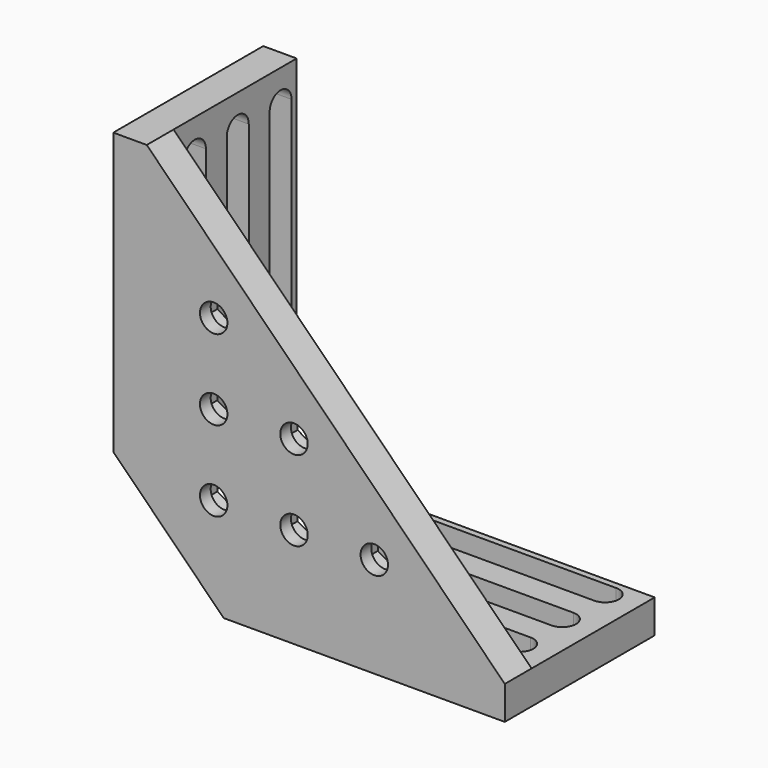
from build123d import *

# Parameters (mm, degrees)
F0_W      = 42
F0_H      = 23
F1_DEPTH  = 5
F3_ANGLE  = 90
F8_R      = 2.05
F9_DEPTH  = 5
F10_DEPTH = 3


# Not quite as in the source:
# - a feature names something its author has since deleted; it is built from what else it names


with BuildPart() as f1:
    # F0 (on Top) → F1 (new body)
    with BuildSketch(Plane.XY):
        Rectangle(F0_W, F0_H)
        with BuildLine():
            ThreePointArc((-16, -9.55), (-18.05, -7.5), (-16, -5.45))
            Line((-16, -5.45), (16, -5.45))
            ThreePointArc((16, -5.45), (18.05, -7.5), (16, -9.55))
            Line((16, -9.55), (-16, -9.55))
        make_face(mode=Mode.SUBTRACT)
        with BuildLine():
            Line((0, -1.55), (-16, -1.55))
            ThreePointArc((-16, -1.55), (-18.05, 0.5), (-16, 2.55))
            Line((-16, 2.55), (0, 2.55))
            Line((0, 2.55), (16, 2.55))
            ThreePointArc((16, 2.55), (18.05, 0.5), (16, -1.55))
            Line((16, -1.55), (0, -1.55))
        make_face(mode=Mode.SUBTRACT)
        with BuildLine():
            Line((16, 6.45), (-16, 6.45))
            ThreePointArc((-16, 6.45), (-18.05, 8.5), (-16, 10.55))
            Line((-16, 10.55), (16, 10.55))
            ThreePointArc((16, 10.55), (18.05, 8.5), (16, 6.45))
        make_face(mode=Mode.SUBTRACT)
    extrude(amount=F1_DEPTH)


with BuildPart() as f3_1:
    # F3: copy of F1
    add(f1.part.rotate(Axis((-21, 0, 2.5), (0, -1, 0)), F3_ANGLE))


with BuildPart() as f3_1_1:
    # F4: moved
    add(f3_1.part.moved(Location((0, 0, 14))))


with BuildPart() as f3_1_2:
    # F5: moved
    add(f3_1_1.part.moved(Location((-14, 0, 0))))


with BuildPart() as f1_1:
    add(f1.part)

    add(f3_1_2.part)  # F9 merges F3_1
    # F8 (on 3pt) → F9 (join)
    with BuildSketch(Plane.XZ.offset(11.5)):
        Polygon((-37.5, 16.5), (-21, 0), (21, 0), (21, 5), (14.4509618943, 11.5490381057), (13.5, 11), (10.0358983849, 13), (10.0358983849, 15.9641016151), (2.4509618943, 23.5490381057), (1.5, 23), (-1.9641016151, 25), (-1.9641016151, 27.9641016151), (-9.5490381057, 35.5490381057), (-10.5, 35), (-13.9641016151, 37), (-13.9641016151, 39.9641016151), (-21.5490381057, 47.5490381057), (-22.5, 47), (-25.9641016151, 49), (-25.9641016151, 51.9641016151), (-32.5, 58.5), (-37.5, 58.5), align=None)
        Polygon((-25.9641016151, 17), (-22.5, 19), (-19.0358983849, 17), (-19.0358983849, 13), (-22.5, 11), (-25.9641016151, 13), align=None, mode=Mode.SUBTRACT)
        Polygon((-13.9641016151, 13), (-13.9641016151, 17), (-10.5, 19), (-7.0358983849, 17), (-7.0358983849, 13), (-10.5, 11), align=None, mode=Mode.SUBTRACT)
        Polygon((-25.9641016151, 25), (-25.9641016151, 29), (-22.5, 31), (-19.0358983849, 29), (-19.0358983849, 25), (-22.5, 23), align=None, mode=Mode.SUBTRACT)
        Polygon((-13.9641016151, 25), (-13.9641016151, 29), (-10.5, 31), (-7.0358983849, 29), (-7.0358983849, 25), (-10.5, 23), align=None, mode=Mode.SUBTRACT)
        Polygon((-1.9641016151, 13), (-1.9641016151, 17), (1.5, 19), (4.9641016151, 17), (4.9641016151, 13), (1.5, 11), align=None, mode=Mode.SUBTRACT)
        Polygon((-25.9641016151, 37), (-25.9641016151, 41), (-22.5, 43), (-19.0358983849, 41), (-19.0358983849, 37), (-22.5, 35), align=None, mode=Mode.SUBTRACT)
        with BuildLine():
            Line((13.5, 11), (14.4509618943, 11.5490381057))
            Line((14.4509618943, 11.5490381057), (12.9839959128, 13.0160040872))
            ThreePointArc((12.9839959128, 13.0160040872), (12.0504310986, 13.5504310986), (11.5160040872, 14.4839959128))
            Line((11.5160040872, 14.4839959128), (10.0358983849, 15.9641016151))
            Line((10.0358983849, 15.9641016151), (10.0358983849, 13))
            Line((10.0358983849, 13), (13.5, 11))
        make_face()
        with BuildLine():
            Line((-24.4839959128, 50.4839959128), (-25.9641016151, 51.9641016151))
            Line((-25.9641016151, 51.9641016151), (-25.9641016151, 49))
            Line((-25.9641016151, 49), (-22.5, 47))
            Line((-22.5, 47), (-21.5490381057, 47.5490381057))
            Line((-21.5490381057, 47.5490381057), (-23.0160040872, 49.0160040872))
            ThreePointArc((-23.0160040872, 49.0160040872), (-23.9495689014, 49.5504310986), (-24.4839959128, 50.4839959128))
        make_face()
        with BuildLine():
            ThreePointArc((11.5160040872, 14.4839959128), (12.0504310986, 13.5504310986), (12.9839959128, 13.0160040872))
            Line((12.9839959128, 13.0160040872), (11.5160040872, 14.4839959128))
        make_face()
        with BuildLine():
            Line((-23.0160040872, 49.0160040872), (-24.4839959128, 50.4839959128))
            ThreePointArc((-24.4839959128, 50.4839959128), (-23.9495689014, 49.5504310986), (-23.0160040872, 49.0160040872))
        make_face()
        with BuildLine():
            Line((1.5, 23), (2.4509618943, 23.5490381057))
            Line((2.4509618943, 23.5490381057), (0.9839959128, 25.0160040872))
            ThreePointArc((0.9839959128, 25.0160040872), (0.0504310986, 25.5504310986), (-0.4839959128, 26.4839959128))
            Line((-0.4839959128, 26.4839959128), (-1.9641016151, 27.9641016151))
            Line((-1.9641016151, 27.9641016151), (-1.9641016151, 25))
            Line((-1.9641016151, 25), (1.5, 23))
        make_face()
        with BuildLine():
            Line((-12.4839959128, 38.4839959128), (-13.9641016151, 39.9641016151))
            Line((-13.9641016151, 39.9641016151), (-13.9641016151, 37))
            Line((-13.9641016151, 37), (-10.5, 35))
            Line((-10.5, 35), (-9.5490381057, 35.5490381057))
            Line((-9.5490381057, 35.5490381057), (-11.0160040872, 37.0160040872))
            ThreePointArc((-11.0160040872, 37.0160040872), (-11.9495689014, 37.5504310986), (-12.4839959128, 38.4839959128))
        make_face()
        with BuildLine():
            ThreePointArc((-0.4839959128, 26.4839959128), (0.0504310986, 25.5504310986), (0.9839959128, 25.0160040872))
            Line((0.9839959128, 25.0160040872), (-0.4839959128, 26.4839959128))
        make_face()
        with BuildLine():
            Line((-11.0160040872, 37.0160040872), (-12.4839959128, 38.4839959128))
            ThreePointArc((-12.4839959128, 38.4839959128), (-11.9495689014, 37.5504310986), (-11.0160040872, 37.0160040872))
        make_face()
        Polygon((-10.5, 31), (-13.9641016151, 29), (-13.9641016151, 25), (-10.5, 23), (-7.0358983849, 25), (-7.0358983849, 29), align=None)
        with Locations((-10.5, 27)):
            Circle(F8_R, mode=Mode.SUBTRACT)
        Polygon((-22.5, 31), (-25.9641016151, 29), (-25.9641016151, 25), (-22.5, 23), (-19.0358983849, 25), (-19.0358983849, 29), align=None)
        with Locations((-22.5, 27)):
            Circle(F8_R, mode=Mode.SUBTRACT)
        Polygon((-22.5, 43), (-25.9641016151, 41), (-25.9641016151, 37), (-22.5, 35), (-19.0358983849, 37), (-19.0358983849, 41), align=None)
        with Locations((-22.5, 39)):
            Circle(F8_R, mode=Mode.SUBTRACT)
        Polygon((-10.5, 19), (-13.9641016151, 17), (-13.9641016151, 13), (-10.5, 11), (-7.0358983849, 13), (-7.0358983849, 17), align=None)
        with Locations((-10.5, 15)):
            Circle(F8_R, mode=Mode.SUBTRACT)
        Polygon((1.5, 19), (-1.9641016151, 17), (-1.9641016151, 13), (1.5, 11), (4.9641016151, 13), (4.9641016151, 17), align=None)
        with Locations((1.5, 15)):
            Circle(F8_R, mode=Mode.SUBTRACT)
        Polygon((-19.0358983849, 17), (-22.5, 19), (-25.9641016151, 17), (-25.9641016151, 13), (-22.5, 11), (-19.0358983849, 13), align=None)
        with Locations((-22.5, 15)):
            Circle(F8_R, mode=Mode.SUBTRACT)
    extrude(amount=F9_DEPTH)

    # F8 (on 3pt) → F10 (cut)
    with BuildSketch(Plane.XZ.offset(11.5)):
        Polygon((-10.5, 31), (-13.9641016151, 29), (-13.9641016151, 25), (-10.5, 23), (-7.0358983849, 25), (-7.0358983849, 29), align=None)
        with Locations((-10.5, 27)):
            Circle(F8_R, mode=Mode.SUBTRACT)
        Polygon((-22.5, 31), (-25.9641016151, 29), (-25.9641016151, 25), (-22.5, 23), (-19.0358983849, 25), (-19.0358983849, 29), align=None)
        with Locations((-22.5, 27)):
            Circle(F8_R, mode=Mode.SUBTRACT)
        Polygon((-22.5, 43), (-25.9641016151, 41), (-25.9641016151, 37), (-22.5, 35), (-19.0358983849, 37), (-19.0358983849, 41), align=None)
        with Locations((-22.5, 39)):
            Circle(F8_R, mode=Mode.SUBTRACT)
        Polygon((-10.5, 19), (-13.9641016151, 17), (-13.9641016151, 13), (-10.5, 11), (-7.0358983849, 13), (-7.0358983849, 17), align=None)
        with Locations((-10.5, 15)):
            Circle(F8_R, mode=Mode.SUBTRACT)
        Polygon((1.5, 19), (-1.9641016151, 17), (-1.9641016151, 13), (1.5, 11), (4.9641016151, 13), (4.9641016151, 17), align=None)
        with Locations((1.5, 15)):
            Circle(F8_R, mode=Mode.SUBTRACT)
        with BuildLine():
            Line((0.9839959128, 25.0160040872), (2.4509618943, 23.5490381057))
            Line((2.4509618943, 23.5490381057), (4.9641016151, 25))
            Line((4.9641016151, 25), (4.9641016151, 29))
            Line((4.9641016151, 29), (1.5, 31))
            Line((1.5, 31), (-1.9641016151, 29))
            Line((-1.9641016151, 29), (-1.9641016151, 27.9641016151))
            Line((-1.9641016151, 27.9641016151), (-0.4839959128, 26.4839959128))
            ThreePointArc((-0.4839959128, 26.4839959128), (1.2398958105, 29.0334320275), (3.55, 27))
            ThreePointArc((3.55, 27), (2.7539321396, 25.3782249881), (0.9839959128, 25.0160040872))
        make_face()
        with BuildLine():
            Line((12.9839959128, 13.0160040872), (14.4509618943, 11.5490381057))
            Line((14.4509618943, 11.5490381057), (16.9641016151, 13))
            Line((16.9641016151, 13), (16.9641016151, 17))
            Line((16.9641016151, 17), (13.5, 19))
            Line((13.5, 19), (10.0358983849, 17))
            Line((10.0358983849, 17), (10.0358983849, 15.9641016151))
            Line((10.0358983849, 15.9641016151), (11.5160040872, 14.4839959128))
            ThreePointArc((11.5160040872, 14.4839959128), (13.2398958105, 17.0334320275), (15.55, 15))
            ThreePointArc((15.55, 15), (14.7539321396, 13.3782249881), (12.9839959128, 13.0160040872))
        make_face()
        Polygon((-19.0358983849, 17), (-22.5, 19), (-25.9641016151, 17), (-25.9641016151, 13), (-22.5, 11), (-19.0358983849, 13), align=None)
        with Locations((-22.5, 15)):
            Circle(F8_R, mode=Mode.SUBTRACT)
    extrude(amount=F10_DEPTH, mode=Mode.SUBTRACT)


solid = f1_1.part
